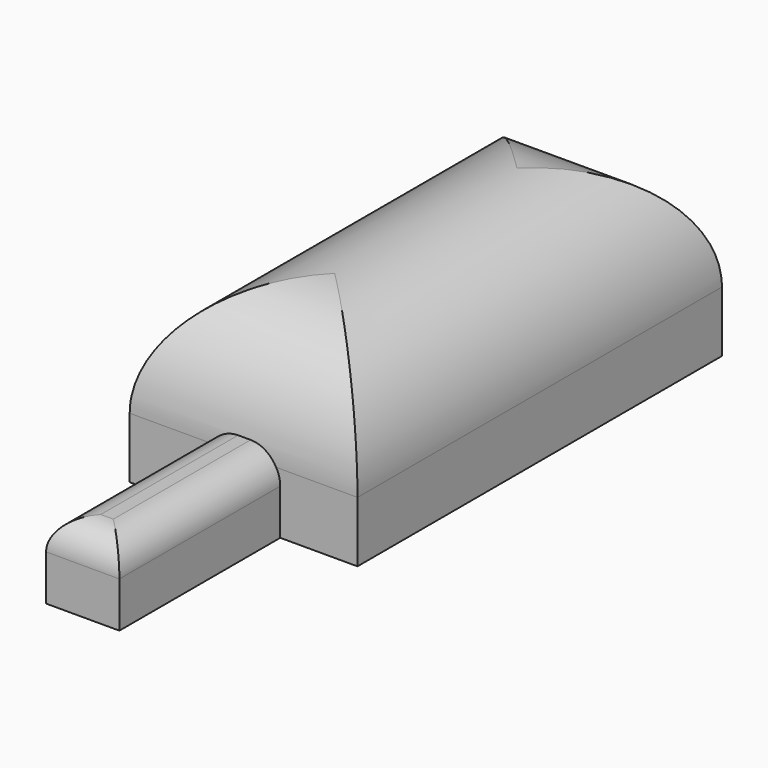
from build123d import *

# Parameters (mm, degrees)
F0_W         = 30
F0_H         = 60
F2_DEPTH     = 23
F3_DEPTH     = 10
F4_T1_DEPTH  = 135
F4_T3_DEPTH  = 105
F4_T8_DEPTH  = 105
F4_T14_DEPTH = 105
F4_T20_DEPTH = 105
F4_T27_DEPTH = 105
F4_T33_DEPTH = 105
F5_R         = 4


# Not quite as in the source:
# - a fillet or chamfer that OpenCascade refuses, or shapes differently, is made with other operations: its cross-section is extruded or revolved along the edge and cut away or added


with BuildPart() as f2:
    # F0 (on Top) → F2 (new body)
    with BuildSketch(Plane.XY):
        Rectangle(F0_W, F0_H)
    extrude(amount=F2_DEPTH)

    # F1 (on face) → F3 (join)
    with BuildSketch(Plane.XY):
        Polygon((4.8278798349, -30), (-4.8278798349, -30), (-4.8278798349, -56.4796291292), (0, -56.4796291292), (4.8278798349, -56.4796291292), align=None)
    extrude(amount=F3_DEPTH)

    # F4: fillet of radius 15 on 4 edges, made by hand

    # F4_s2 → F4_t1 (cut)
    with BuildSketch(Plane.XZ.offset(-67.5)):
        with BuildLine():
            ThreePointArc((-15, 8), (-10.6066017178, 18.6066017178), (0, 23))
            Line((0, 23), (-15, 23))
            Line((-15, 23), (-15, 8))
        make_face()
        with BuildLine():
            ThreePointArc((15, 8), (10.6066017178, 18.6066017178), (0, 23))
            Line((0, 23), (15, 23))
            Line((15, 23), (15, 8))
        make_face()
    extrude(amount=F4_T1_DEPTH, mode=Mode.SUBTRACT)

    # F4_s4 → F4_t3 (cut)
    with BuildSketch(Plane.YZ.offset(-52.5)):
        with BuildLine():
            ThreePointArc((30, 8), (25.6066017178, 18.6066017178), (15, 23))
            Line((15, 23), (30, 23))
            Line((30, 23), (30, 8))
        make_face()
    extrude(amount=F4_T3_DEPTH, mode=Mode.SUBTRACT)


with BuildPart() as f4_tool6:
    # F4_s7 → F4_t8 (new body)
    with BuildSketch(Plane.YZ.offset(-52.5)):
        with BuildLine():
            ThreePointArc((-15, 23), (-25.6066017178, 18.6066017178), (-30, 8))
            Line((-30, 8), (-30, 23))
            Line((-30, 23), (-15, 23))
        make_face()
    extrude(amount=F4_T8_DEPTH)

    split(bisect_by=Plane.YZ.offset(-4.8278798349), keep=Keep.BOTTOM)

    split(bisect_by=Plane.XY.offset(10), keep=Keep.TOP)


with BuildPart() as f2_1:
    add(f2.part)

    # F4_t5: cut F4_tool6
    add(f4_tool6.part, mode=Mode.SUBTRACT)


with BuildPart() as f4_tool12:
    # F4_s13 → F4_t14 (new body)
    with BuildSketch(Plane.YZ.offset(-52.5)):
        with BuildLine():
            ThreePointArc((-15, 23), (-25.6066017178, 18.6066017178), (-30, 8))
            Line((-30, 8), (-30, 23))
            Line((-30, 23), (-15, 23))
        make_face()
    extrude(amount=F4_T14_DEPTH)

    split(bisect_by=Plane.YZ.offset(-4.8278798349), keep=Keep.BOTTOM)

    split(bisect_by=Plane.XY.offset(10), keep=Keep.BOTTOM)


with BuildPart() as f2_2:
    add(f2_1.part)

    # F4_t11: cut F4_tool12
    add(f4_tool12.part, mode=Mode.SUBTRACT)


with BuildPart() as f4_tool18:
    # F4_s19 → F4_t20 (new body)
    with BuildSketch(Plane.YZ.offset(-52.5)):
        with BuildLine():
            ThreePointArc((-15, 23), (-25.6066017178, 18.6066017178), (-30, 8))
            Line((-30, 8), (-30, 23))
            Line((-30, 23), (-15, 23))
        make_face()
    extrude(amount=F4_T20_DEPTH)

    split(bisect_by=Plane.YZ.offset(-4.8278798349), keep=Keep.TOP)

    split(bisect_by=Plane.XY.offset(10), keep=Keep.TOP)

    split(bisect_by=Plane.YZ.offset(4.8278798349), keep=Keep.BOTTOM)


with BuildPart() as f2_3:
    add(f2_2.part)

    # F4_t17: cut F4_tool18
    add(f4_tool18.part, mode=Mode.SUBTRACT)


with BuildPart() as f4_tool25:
    # F4_s26 → F4_t27 (new body)
    with BuildSketch(Plane.YZ.offset(-52.5)):
        with BuildLine():
            ThreePointArc((-15, 23), (-25.6066017178, 18.6066017178), (-30, 8))
            Line((-30, 8), (-30, 23))
            Line((-30, 23), (-15, 23))
        make_face()
    extrude(amount=F4_T27_DEPTH)

    split(bisect_by=Plane.XY.offset(10), keep=Keep.TOP)

    split(bisect_by=Plane.YZ.offset(4.8278798349), keep=Keep.TOP)


with BuildPart() as f2_4:
    add(f2_3.part)

    # F4_t24: cut F4_tool25
    add(f4_tool25.part, mode=Mode.SUBTRACT)


with BuildPart() as f4_tool31:
    # F4_s32 → F4_t33 (new body)
    with BuildSketch(Plane.YZ.offset(-52.5)):
        with BuildLine():
            ThreePointArc((-15, 23), (-25.6066017178, 18.6066017178), (-30, 8))
            Line((-30, 8), (-30, 23))
            Line((-30, 23), (-15, 23))
        make_face()
    extrude(amount=F4_T33_DEPTH)

    split(bisect_by=Plane.XY.offset(10), keep=Keep.BOTTOM)

    split(bisect_by=Plane.YZ.offset(4.8278798349), keep=Keep.TOP)


with BuildPart() as f2_5:
    add(f2_4.part)

    # F4_t30: cut F4_tool31
    add(f4_tool31.part, mode=Mode.SUBTRACT)

    # F5
    f5_edges = [f2_5.edges().sort_by_distance(p)[0] for p in [
        (-4.82788, -43.172849, 10),
        (4.82788, -43.172849, 10),
        (0, -56.479629, 10),
    ]]
    fillet(f5_edges, radius=F5_R)


solid = f2_5.part
